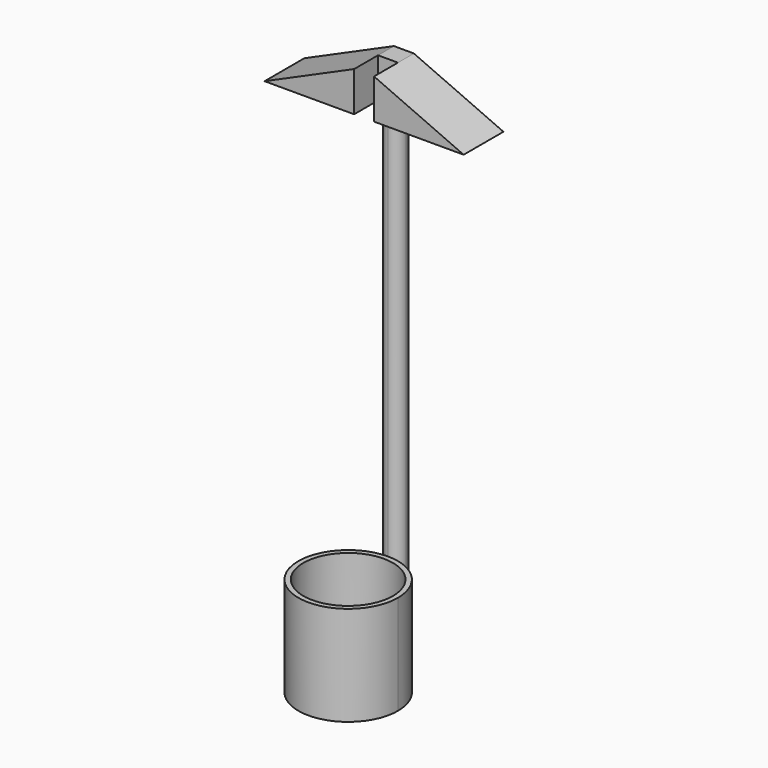
from build123d import *

# Parameters (mm, degrees)
F0_R     = 22.5
F1_DEPTH = 50
F2_DEPTH = 250
F3_DEPTH = 5
F5_DEPTH = 20
F7_DEPTH = 25


with BuildPart() as f1:
    # F0 (on Top) → F1 (new body)
    with BuildSketch(Plane.XY):
        with BuildLine():
            ThreePointArc((0, 25), (-17.6776695297, -17.6776695297), (25, 0))
            ThreePointArc((25, 0), (17.6776695297, 17.6776695297), (0, 25))
        make_face()
        Circle(F0_R, mode=Mode.SUBTRACT)
    extrude(amount=F1_DEPTH)

    # F0 (on Top) → F3 (join)
    with BuildSketch(Plane.XY):
        Circle(F0_R)
    extrude(amount=F3_DEPTH)


with BuildPart() as f2:
    # F0 (on Top) → F2 (new body)
    with BuildSketch(Plane.XY):
        with BuildLine():
            ThreePointArc((5, 30), (-3.5355339059, 33.5355339059), (0, 25))
            ThreePointArc((0, 25), (3.5355339059, 26.4644660941), (5, 30))
        make_face()
    extrude(amount=F2_DEPTH)

    # F4 (on face) → F5 (join)
    with BuildSketch(Plane.XY.offset(250)):
        with BuildLine():
            Line((0, 35), (-5, 35))
            Line((-5, 35), (-5, 30))
            ThreePointArc((-5, 30), (-3.5355339059, 33.5355339059), (0, 35))
        make_face()
        with BuildLine():
            ThreePointArc((5, 30), (3.5355339059, 33.5355339059), (0, 35))
            ThreePointArc((0, 35), (-3.5355339059, 33.5355339059), (-5, 30))
            ThreePointArc((-5, 30), (-3.5355339059, 26.4644660941), (0, 25))
            ThreePointArc((0, 25), (3.5355339059, 26.4644660941), (5, 30))
        make_face()
        with BuildLine():
            Line((5, 35), (0, 35))
            ThreePointArc((0, 35), (3.5355339059, 33.5355339059), (5, 30))
            Line((5, 30), (5, 35))
        make_face()
        with BuildLine():
            Line((5, 25), (5, 30))
            ThreePointArc((5, 30), (3.5355339059, 26.4644660941), (0, 25))
            Line((0, 25), (5, 25))
        make_face()
        with BuildLine():
            ThreePointArc((0, 25), (-3.5355339059, 26.4644660941), (-5, 30))
            Line((-5, 30), (-5, 25))
            Line((-5, 25), (0, 25))
        make_face()
    extrude(amount=F5_DEPTH)


with BuildPart() as f7:
    # F6 (on face) → F7 (new body)
    with BuildSketch(Plane(origin=(0, 35, 0), x_dir=(-1, 0, 0), z_dir=(0, 1, 0))):
        Polygon((-50, 250), (-5, 250), (-5, 270), align=None)
    extrude(amount=-F7_DEPTH)


with BuildPart() as f7b:
    # F6 (on face) → F7, piece 2 (new body)
    with BuildSketch(Plane(origin=(0, 35, 0), x_dir=(-1, 0, 0), z_dir=(0, 1, 0))):
        Polygon((5, 270), (5, 250), (50, 250), align=None)
    extrude(amount=-F7_DEPTH)


solid = Compound([f1.part, f2.part, f7.part, f7b.part])
